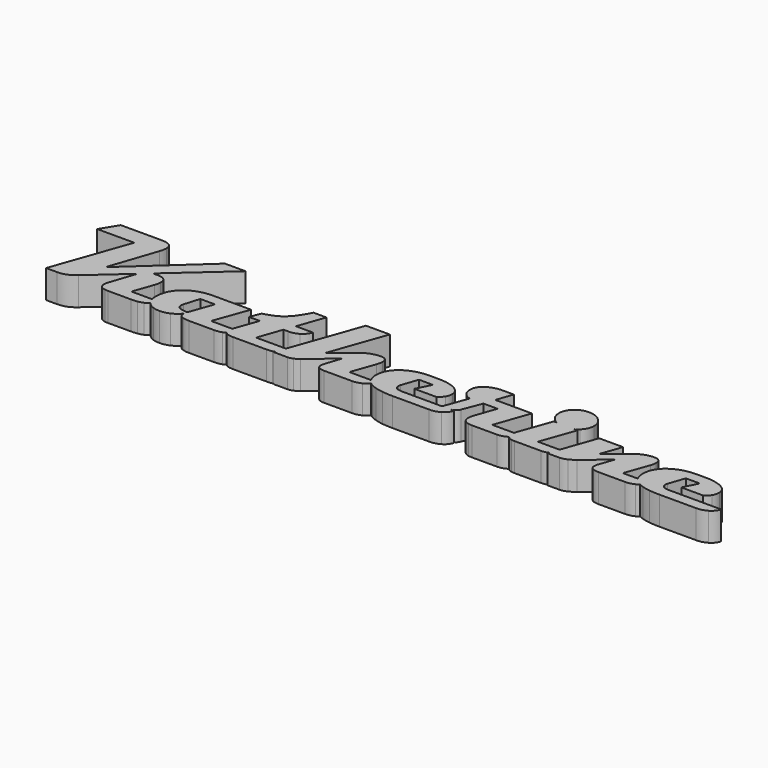
from build123d import *

# Parameters (mm, degrees)
F1_DEPTH = 5


# Not quite as in the source:
# - ends of sketch curves that miss each other by under 0.0002 mm in the source are joined


with BuildPart() as f1:
    # F0 (on Top) → F1 (new body)
    with BuildSketch(Plane.XY):
        with BuildLine():
            ThreePointArc((-41.0388538913, -7.7829862783), (-40.6519052256, -7.5879306027), (-40.3085009865, -7.3236400145))
            ThreePointArc((-40.3085009865, -7.3236400145), (-40.22279605, -7.4225124425), (-40.132811973, -7.5175069733))
            ThreePointArc((-40.132811973, -7.5175069733), (-39.6547267524, -7.8982007095), (-39.1054880503, -8.1662121401))
            ThreePointArc((-39.1054880503, -8.1662121401), (-38.514353508, -8.3159016782), (-37.9062499945, -8.3612574439))
            ThreePointArc((-37.9062499945, -8.3612574439), (-37.0183057676, -8.2719267598), (-36.171682056, -7.9896978786))
            ThreePointArc((-36.171682056, -7.9896978786), (-35.4124918652, -7.5219262203), (-34.7656252151, -6.9081318158))
            ThreePointArc((-34.7656252151, -6.9081318158), (-34.5927962521, -7.5326313151), (-34.0823731355, -7.9318023768))
            ThreePointArc((-34.0823731355, -7.9318023768), (-33.484211348, -8.0880881874), (-32.867187983, -8.1268825052))
            Line((-32.867187983, -8.1268825052), (-28.425781, -8.126882))
            ThreePointArc((-28.425781, -8.126882), (-27.7355719457, -8.079447321), (-27.0641798893, -7.9125003217))
            ThreePointArc((-27.0641798893, -7.9125003217), (-26.7952592168, -7.7985265504), (-26.5427710109, -7.6516999837))
            ThreePointArc((-26.5427710109, -7.6516999837), (-26.3855476723, -7.8009864955), (-26.2007460852, -7.9143621784))
            ThreePointArc((-26.2007460852, -7.9143621784), (-25.6396105798, -8.0847606699), (-25.0546880158, -8.1268816008))
            Line((-25.0546880158, -8.1268816008), (-19.078125, -8.126882))
            ThreePointArc((-19.078125, -8.126882), (-18.611136062, -8.1073181164), (-18.1483309647, -8.0419511841))
            ThreePointArc((-18.1483309647, -8.0419511841), (-17.9537595174, -7.9983783321), (-17.7625579106, -7.9418222687))
            Line((-17.7625579106, -7.9418222687), (-17.828125, -8.126882))
            Line((-17.828125, -8.126882), (-15.414062, -8.126882))
            ThreePointArc((-15.414062, -8.126882), (-14.9371612708, -8.0768882377), (-14.4806716144, -7.9300858764))
            ThreePointArc((-14.4806716144, -7.9300858764), (-14.0602330965, -7.7019026098), (-13.6796876954, -7.4120383418))
            Line((-13.6796876954, -7.4120383418), (-9.238281, -3.755788))
            Line((-9.238281, -3.755788), (-10.082031, -6.251882))
            ThreePointArc((-10.082031, -6.251882), (-10.2043236485, -6.7022972187), (-10.2578121557, -7.1659439938))
            ThreePointArc((-10.2578121557, -7.1659439938), (-10.1557870737, -7.6253643767), (-9.8188523394, -7.953923647))
            ThreePointArc((-9.8188523394, -7.953923647), (-9.3864269164, -8.0926292054), (-8.9335939926, -8.1268821757))
            Line((-8.9335939926, -8.1268821757), (-3.941406, -8.126882))
            ThreePointArc((-3.941406, -8.126882), (-3.1533912263, -8.0403408721), (-2.40624961, -7.7753197938))
            ThreePointArc((-2.40624961, -7.7753197938), (-1.8869380355, -7.4484134341), (-1.4674728436, -7.0005281127))
            ThreePointArc((-1.4674728436, -7.0005281127), (-1.2242477019, -7.1810316698), (-0.963881859, -7.3357887326))
            ThreePointArc((-0.963881859, -7.3357887326), (-0.4833529132, -7.5654364797), (0.0188309888, -7.7427990379))
            ThreePointArc((0.0188309888, -7.7427990379), (0.6955627885, -7.9114479696), (1.3839819805, -8.0231951624))
            ThreePointArc((1.3839819805, -8.0231951624), (2.2860736975, -8.1032829505), (3.1914060019, -8.1268823587))
            Line((3.1914060019, -8.1268823587), (9.71875, -8.126882))
            ThreePointArc((9.71875, -8.126882), (10.6459551299, -8.0188860378), (11.5117191005, -7.6698511769))
            ThreePointArc((11.5117191005, -7.6698511769), (12.2182935812, -7.0751735424), (12.636719156, -6.2518820431))
            Line((12.636719156, -6.2518820431), (11.839904, -6.251882))
            ThreePointArc((11.839904, -6.251882), (12.2203316946, -6.1982560334), (12.5803771638, -6.0642103268))
            ThreePointArc((12.5803771638, -6.0642103268), (12.9236125857, -5.781978222), (13.1445308052, -5.3964129313))
            Line((13.1445308052, -5.3964129313), (14.445312, -2.033132))
            Line((14.445312, -2.033132), (16.941406, -2.033132))
            Line((16.941406, -2.033132), (15.617188, -5.841726))
            ThreePointArc((15.617188, -5.841726), (15.5069945684, -6.2396126308), (15.4648440894, -6.6503190016))
            ThreePointArc((15.4648440894, -6.6503190016), (15.5249861611, -7.1431102722), (15.7443677625, -7.5884551717))
            ThreePointArc((15.7443677625, -7.5884551717), (16.1291631955, -7.9030957183), (16.5985890064, -8.0665139602))
            ThreePointArc((16.5985890064, -8.0665139602), (16.9207946447, -8.1132894302), (17.2460940026, -8.1268822795))
            Line((17.2460940026, -8.1268822795), (21.734375, -8.126882))
            ThreePointArc((21.734375, -8.126882), (22.6012721335, -7.9986668615), (23.3984381814, -7.6346942836))
            ThreePointArc((23.3984381814, -7.6346942836), (23.4163816488, -7.6239283489), (23.4342230306, -7.6129940494))
            ThreePointArc((23.4342230306, -7.6129940494), (23.7939058179, -7.9122336142), (24.2348819523, -8.0686182877))
            ThreePointArc((24.2348819523, -8.0686182877), (24.5397453002, -8.1137749766), (24.847655998, -8.1268817965))
            Line((24.847655998, -8.1268817965), (29.476562, -8.126882))
            ThreePointArc((29.476562, -8.126882), (30.1070405693, -8.0706131317), (30.7147858815, -7.8936527037))
            Line((30.7147858815, -7.8936527037), (30.632812, -8.126882))
            Line((30.632812, -8.126882), (32.789062, -8.126882))
            ThreePointArc((32.789062, -8.126882), (33.4235776604, -8.0266967564), (34.0223620143, -7.7940930276))
            ThreePointArc((34.0223620143, -7.7940930276), (34.5848534171, -7.4904326401), (35.1210935284, -7.1425063335))
            Line((35.1210935284, -7.1425063335), (39.152344, -3.732351))
            Line((39.152344, -3.732351), (38.261719, -6.251882))
            ThreePointArc((38.261719, -6.251882), (38.1461449931, -6.6553294459), (38.0976563403, -7.0721940116))
            ThreePointArc((38.0976563403, -7.0721940116), (38.2393214885, -7.6057214469), (38.6672498677, -7.9544303412))
            ThreePointArc((38.6672498677, -7.9544303412), (39.1765365419, -8.0926198874), (39.7031250191, -8.1268825466))
            Line((39.7031250191, -8.1268825466), (44.378906, -8.126882))
            ThreePointArc((44.378906, -8.126882), (45.1897724676, -8.0404274116), (45.9609379296, -7.7753188519))
            ThreePointArc((45.9609379296, -7.7753188519), (46.2492028992, -7.6272789388), (46.5147649013, -7.4415658775))
            ThreePointArc((46.5147649013, -7.4415658775), (46.8972420105, -7.6083787214), (47.2922689888, -7.7427990379))
            ThreePointArc((47.2922689888, -7.7427990379), (47.9690007885, -7.9114479696), (48.6574199805, -8.0231951624))
            ThreePointArc((48.6574199805, -8.0231951624), (49.5595116975, -8.1032829505), (50.4648440019, -8.1268823587))
            Line((50.4648440019, -8.1268823587), (56.992188, -8.126882))
            ThreePointArc((56.992188, -8.126882), (57.9193926144, -8.0188859143), (58.7851561005, -7.6698511769))
            ThreePointArc((58.7851561005, -7.6698511769), (59.4917305812, -7.0751735424), (59.910156156, -6.2518820431))
            Line((59.910156156, -6.2518820431), (50.769531, -6.251882))
            ThreePointArc((50.769531, -6.251882), (50.2800688414, -6.2224290609), (49.8042389453, -6.1039951567))
            ThreePointArc((49.8042389453, -6.1039951567), (49.3904767485, -5.7971432464), (49.2460942663, -5.3026630107))
            ThreePointArc((49.2460942663, -5.3026630107), (49.2694447459, -5.0767529806), (49.3281248503, -4.857350947))
            Line((49.3281248503, -4.857350947), (50.289062, -2.033132))
            Line((50.289062, -2.033132), (52.761719, -2.033132))
            Line((52.761719, -2.033132), (51.496094, -4.552663))
            Line((51.496094, -4.552663), (55.375, -4.552663))
            ThreePointArc((55.375, -4.552663), (55.8700343287, -4.1640167477), (56.2711331062, -3.6790170702))
            ThreePointArc((56.2711331062, -3.6790170702), (56.5212419766, -3.0971474905), (56.5820304087, -2.4667260348))
            ThreePointArc((56.5820304087, -2.4667260348), (56.4379602582, -1.8376863502), (56.0804739077, -1.3004240892))
            ThreePointArc((56.0804739077, -1.3004240892), (55.5823321611, -0.901279248), (55.0117188478, -0.6151634052))
            ThreePointArc((55.0117188478, -0.6151634052), (53.7271032287, -0.2607110717), (52.398438, -0.1581319954))
            Line((52.398438, -0.1581319954), (50.699219, -0.158132))
            ThreePointArc((50.699219, -0.158132), (49.655951865, -0.2168728292), (48.6284059644, -0.4066258583))
            ThreePointArc((48.6284059644, -0.4066258583), (47.6382703006, -0.7445081432), (46.7148434962, -1.2362562132))
            ThreePointArc((46.7148434962, -1.2362562132), (45.9049173012, -1.8810517052), (45.2715183551, -2.6999212121))
            ThreePointArc((45.2715183551, -2.6999212121), (44.8881179339, -3.6632607226), (44.7695312778, -4.6932879952))
            ThreePointArc((44.7695312778, -4.6932879952), (44.8572165929, -5.4925155477), (45.151179856, -6.24087308))
            ThreePointArc((45.151179856, -6.24087308), (45.154501283, -6.2463809553), (45.1578343541, -6.2518817849))
            Line((45.1578343541, -6.2518817849), (42.515625, -6.251882))
            Line((42.515625, -6.251882), (44.027344, -2.033132))
            ThreePointArc((44.027344, -2.033132), (44.1611952062, -1.5545343527), (44.2148435791, -1.0604759891))
            ThreePointArc((44.2148435791, -1.0604759891), (44.1842972495, -0.7081778218), (44.0715740853, -0.3730054344))
            ThreePointArc((44.0715740853, -0.3730054344), (43.8469326529, -0.094309699), (43.5329259746, 0.0775479194))
            ThreePointArc((43.5329259746, 0.0775479194), (43.3025846965, 0.1347784403), (43.0664060133, 0.1582744947))
            ThreePointArc((43.0664060133, 0.1582744947), (42.2122955756, 0.1015966261), (41.3850749029, -0.1184557395))
            ThreePointArc((41.3850749029, -0.1184557395), (40.6142153902, -0.4879783148), (39.9140620054, -0.9784440065))
            Line((39.9140620054, -0.9784440065), (36.339844, -3.908132))
            Line((36.339844, -3.908132), (37.664062, -0.158132))
            Line((37.664062, -0.158132), (33.433594, -0.158132))
            Line((33.433594, -0.158132), (31.29182, -6.251882))
            Line((31.29182, -6.251882), (27.460938, -6.251882))
            Line((27.460938, -6.251882), (29.628906, -0.158132))
            Line((29.628906, -0.158132), (29.101799, -0.158132))
            ThreePointArc((29.101799, -0.158132), (29.4068732284, 0.0364904062), (29.6874191096, 0.2650558804))
            ThreePointArc((29.6874191096, 0.2650558804), (30.366494837, 1.1592707544), (30.6014809526, 2.2572439911))
            ThreePointArc((30.6014809526, 2.2572439911), (30.3650999562, 3.349316412), (29.687419254, 4.2377123016))
            ThreePointArc((29.687419254, 4.2377123016), (28.6767977861, 4.8583731282), (27.5077320018, 5.058024915))
            ThreePointArc((27.5077320018, 5.058024915), (26.3218756584, 4.8596410547), (25.2928876513, 4.2377123876))
            ThreePointArc((25.2928876513, 4.2377123876), (24.6229039835, 3.3471735476), (24.3905443219, 2.2572440024))
            ThreePointArc((24.3905443219, 2.2572440024), (24.6215298062, 1.1614186069), (25.2928885037, 0.2650565856))
            ThreePointArc((25.2928885037, 0.2650565856), (25.5782381644, 0.0364437748), (25.8877997548, -0.1581324447))
            Line((25.8877997548, -0.1581324447), (25.375, -0.158132))
            Line((25.375, -0.158132), (23.335938, -5.865163))
            ThreePointArc((23.335938, -5.865163), (23.2722807861, -6.0563098529), (23.2238976669, -6.2518819314))
            Line((23.2238976669, -6.2518819314), (19.390625, -6.251882))
            Line((19.390625, -6.251882), (21.523438, -0.158132))
            Line((21.523438, -0.158132), (15.042969, -0.158132))
            Line((15.042969, -0.158132), (16.027344, 2.701243))
            Line((16.027344, 2.701243), (14.128906, 2.701243))
            ThreePointArc((14.128906, 2.701243), (12.8459099225, 2.5629289583), (11.6445314146, 2.0918672533))
            ThreePointArc((11.6445314146, 2.0918672533), (11.129729496, 1.7160662558), (10.7202319924, 1.227641005))
            ThreePointArc((10.7202319924, 1.227641005), (10.4686111855, 0.6402086019), (10.3906249833, 0.0059309997))
            ThreePointArc((10.3906249833, 0.0059309997), (10.5009666486, -0.6884259245), (10.8359373198, -1.3065695346))
            ThreePointArc((10.8359373198, -1.3065695346), (11.3648859964, -1.772232468), (12.0195309784, -2.0331321023))
            Line((12.0195309784, -2.0331321023), (10.484375, -6.251882))
            Line((10.484375, -6.251882), (3.496094, -6.251882))
            ThreePointArc((3.496094, -6.251882), (3.006631802, -6.2224292081), (2.5308018367, -6.1039954679))
            ThreePointArc((2.5308018367, -6.1039954679), (2.1170390203, -5.7971436366), (1.9726562663, -5.3026630107))
            ThreePointArc((1.9726562663, -5.3026630107), (1.9960067761, -5.0767528164), (2.0546869618, -4.8573506322))
            Line((2.0546869618, -4.8573506322), (3.015625, -2.033132))
            Line((3.015625, -2.033132), (5.488281, -2.033132))
            Line((5.488281, -2.033132), (4.222656, -4.552663))
            Line((4.222656, -4.552663), (8.101562, -4.552663))
            ThreePointArc((8.101562, -4.552663), (8.5965968277, -4.1640172361), (8.9976958023, -3.6790175301))
            ThreePointArc((8.9976958023, -3.6790175301), (9.2478049105, -3.0971477482), (9.3085934087, -2.4667260348))
            ThreePointArc((9.3085934087, -2.4667260348), (9.1645232582, -1.8376863502), (8.8070369077, -1.3004240892))
            ThreePointArc((8.8070369077, -1.3004240892), (8.30889446, -0.9012794397), (7.7382808478, -0.6151634052))
            ThreePointArc((7.7382808478, -0.6151634052), (6.4536652762, -0.2607109052), (5.1250000003, -0.1581320144))
            Line((5.1250000003, -0.1581320144), (3.425781, -0.158132))
            ThreePointArc((3.425781, -0.158132), (2.3825143466, -0.2168727714), (1.3549689052, -0.4066256223))
            ThreePointArc((1.3549689052, -0.4066256223), (0.3648329143, -0.7445083107), (-0.558594213, -1.2362566674))
            ThreePointArc((-0.558594213, -1.2362566674), (-1.3685205188, -1.8810515227), (-2.001919382, -2.6999207719))
            ThreePointArc((-2.001919382, -2.6999207719), (-2.3853200085, -3.663260494), (-2.5039067219, -4.6932880126))
            ThreePointArc((-2.5039067219, -4.6932880126), (-2.4162214099, -5.4925155365), (-2.122258144, -6.24087308))
            ThreePointArc((-2.122258144, -6.24087308), (-2.1189365827, -6.2463811774), (-2.1156033764, -6.2518822286))
            Line((-2.1156033764, -6.2518822286), (-5.933594, -6.251882))
            Line((-5.933594, -6.251882), (-4.445312, -2.056569))
            ThreePointArc((-4.445312, -2.056569), (-4.2962027253, -1.5677640498), (-4.2343749085, -1.0604760031))
            ThreePointArc((-4.2343749085, -1.0604760031), (-4.264964304, -0.7054373618), (-4.3791526844, -0.367873849))
            ThreePointArc((-4.3791526844, -0.367873849), (-4.6101733479, -0.0900127869), (-4.9328180579, 0.0727067842))
            ThreePointArc((-4.9328180579, 0.0727067842), (-5.167278777, 0.1209568243), (-5.4062499891, 0.1348362469))
            ThreePointArc((-5.4062499891, 0.1348362469), (-7.0783618637, -0.1522624726), (-8.546875426, -1.0018814961))
            Line((-8.546875426, -1.0018814961), (-12.121094, -3.931569))
            Line((-12.121094, -3.931569), (-8.59375, 6.029368))
            Line((-8.59375, 6.029368), (-12.8125, 6.029368))
            Line((-12.8125, 6.029368), (-17.163804, -6.251882))
            Line((-17.163804, -6.251882), (-22.441406, -6.251882))
            Line((-22.441406, -6.251882), (-20.976562, -2.033132))
            Line((-20.976562, -2.033132), (-20.203125, -2.033132))
            ThreePointArc((-20.203125, -2.033132), (-19.2756378797, -1.9378814192), (-18.4071571664, -1.5986967007))
            ThreePointArc((-18.4071571664, -1.5986967007), (-17.7058793456, -0.9769745522), (-17.2499994481, -0.1581321948))
            Line((-17.2499994481, -0.1581321948), (-20.273438, -0.158132))
            Line((-20.273438, -0.158132), (-18.621094, 4.541087))
            Line((-18.621094, 4.541087), (-20.90625, 4.541087))
            ThreePointArc((-20.90625, 4.541087), (-21.4082641486, 3.6355982063), (-21.9586683607, 2.7586812403))
            ThreePointArc((-21.9586683607, 2.7586812403), (-22.5796445291, 1.92765861), (-23.3085938874, 1.1895238724))
            ThreePointArc((-23.3085938874, 1.1895238724), (-24.0054210978, 0.7213318148), (-24.7628910956, 0.3593772445))
            ThreePointArc((-24.7628910956, 0.3593772445), (-25.5502591432, 0.0731695146), (-26.3554690761, -0.1581316958))
            Line((-26.3554690761, -0.1581316958), (-27.09375, -2.033132))
            Line((-27.09375, -2.033132), (-25.171875, -2.033132))
            Line((-25.171875, -2.033132), (-26.660156, -6.251882))
            Line((-26.660156, -6.251882), (-30.417969, -6.251882))
            Line((-30.417969, -6.251882), (-28.214844, -0.158132))
            Line((-28.214844, -0.158132), (-34.90625, -0.158132))
            ThreePointArc((-34.90625, -0.158132), (-36.0221039955, -0.2269664901), (-37.1171681088, -0.4521396119))
            ThreePointArc((-37.1171681088, -0.4521396119), (-38.161317732, -0.8572023125), (-39.1132812218, -1.4471937065))
            ThreePointArc((-39.1132812218, -1.4471937065), (-39.9257194244, -2.2112724829), (-40.531441201, -3.1477409021))
            ThreePointArc((-40.531441201, -3.1477409021), (-40.8817480076, -4.2053613935), (-40.9882812346, -5.3143820038))
            ThreePointArc((-40.9882812346, -5.3143820038), (-40.9691758556, -5.7876744475), (-40.87493104, -6.2518820115))
            Line((-40.87493104, -6.2518820115), (-44.523438, -6.251882))
            Line((-44.523438, -6.251882), (-43.28125, -2.701101))
            ThreePointArc((-43.28125, -2.701101), (-43.1235684428, -2.1596888013), (-43.0585937077, -1.5995380092))
            ThreePointArc((-43.0585937077, -1.5995380092), (-43.1099377226, -1.1346477281), (-43.2992018036, -0.7069348741))
            ThreePointArc((-43.2992018036, -0.7069348741), (-43.6468217868, -0.3901658617), (-44.0856330523, -0.2209712833))
            ThreePointArc((-44.0856330523, -0.2209712833), (-44.3906532486, -0.1722416863), (-44.6992190003, -0.1581319688))
            Line((-44.6992190003, -0.1581319688), (-45.589844, -0.158132))
            Line((-45.589844, -0.158132), (-36.003906, 8.361399))
            Line((-36.003906, 8.361399), (-39.660156, 8.361399))
            Line((-39.660156, 8.361399), (-51.894531, -2.794851))
            Line((-51.894531, -2.794851), (-49.046875, 5.654368))
            ThreePointArc((-49.046875, 5.654368), (-48.8813500977, 6.2425465867), (-48.8125003888, 6.8496810125))
            ThreePointArc((-48.8125003888, 6.8496810125), (-48.8894317366, 7.3840406512), (-49.1628369085, 7.849560081))
            ThreePointArc((-49.1628369085, 7.849560081), (-49.6049665301, 8.153163549), (-50.1192419874, 8.3053950955))
            ThreePointArc((-50.1192419874, 8.3053950955), (-50.4665897561, 8.3487614028), (-50.816405998, 8.3613987474))
            Line((-50.816405998, 8.3613987474), (-58.117188, 8.361399))
            Line((-58.117188, 8.361399), (-59.910156, 5.408274))
            Line((-59.910156, 5.408274), (-53.359375, 5.408274))
            Line((-53.359375, 5.408274), (-58.140625, -8.126882))
            Line((-58.140625, -8.126882), (-56.171875, -8.126882))
            ThreePointArc((-56.171875, -8.126882), (-54.6376955368, -7.8473347977), (-53.3124999078, -7.0253191004))
            Line((-53.3124999078, -7.0253191004), (-47.195312, -1.576101))
            Line((-47.195312, -1.576101), (-48.753906, -6.251882))
            ThreePointArc((-48.753906, -6.251882), (-48.8307742641, -6.5583307959), (-48.859375235, -6.8729759969))
            ThreePointArc((-48.859375235, -6.8729759969), (-48.7932045611, -7.3204003692), (-48.5593058024, -7.7075158189))
            ThreePointArc((-48.5593058024, -7.7075158189), (-48.186140851, -7.9567312154), (-47.7549960724, -8.0811285669))
            ThreePointArc((-47.7549960724, -8.0811285669), (-47.4644203662, -8.1165567713), (-47.1718750003, -8.1268819666))
            Line((-47.1718750003, -8.1268819666), (-43.070312, -8.126882))
            ThreePointArc((-43.070312, -8.126882), (-42.5526130393, -8.1104042475), (-42.0375880961, -8.0553313365))
            ThreePointArc((-42.0375880961, -8.0553313365), (-41.5295966051, -7.9507858889), (-41.0388538913, -7.7829862783))
        make_face()
        with BuildLine():
            Line((-35.703125, -2.033132), (-33.113281, -2.033132))
            Line((-33.113281, -2.033132), (-34.601562, -6.251882))
            ThreePointArc((-34.601562, -6.251882), (-34.9452052027, -6.2435805403), (-35.2877540687, -6.2149476054))
            ThreePointArc((-35.2877540687, -6.2149476054), (-35.6272696166, -6.1579878962), (-35.9570660143, -6.0592480388))
            ThreePointArc((-35.9570660143, -6.0592480388), (-36.1656705705, -5.9584813606), (-36.3511852421, -5.8197222661))
            ThreePointArc((-36.3511852421, -5.8197222661), (-36.5352043133, -5.551944775), (-36.5937497164, -5.2323510083))
            ThreePointArc((-36.5937497164, -5.2323510083), (-36.5740112067, -4.9956634479), (-36.5234372116, -4.7636012269))
            Line((-36.5234372116, -4.7636012269), (-35.703125, -2.033132))
        make_face(mode=Mode.SUBTRACT)
    extrude(amount=F1_DEPTH)


solid = f1.part
